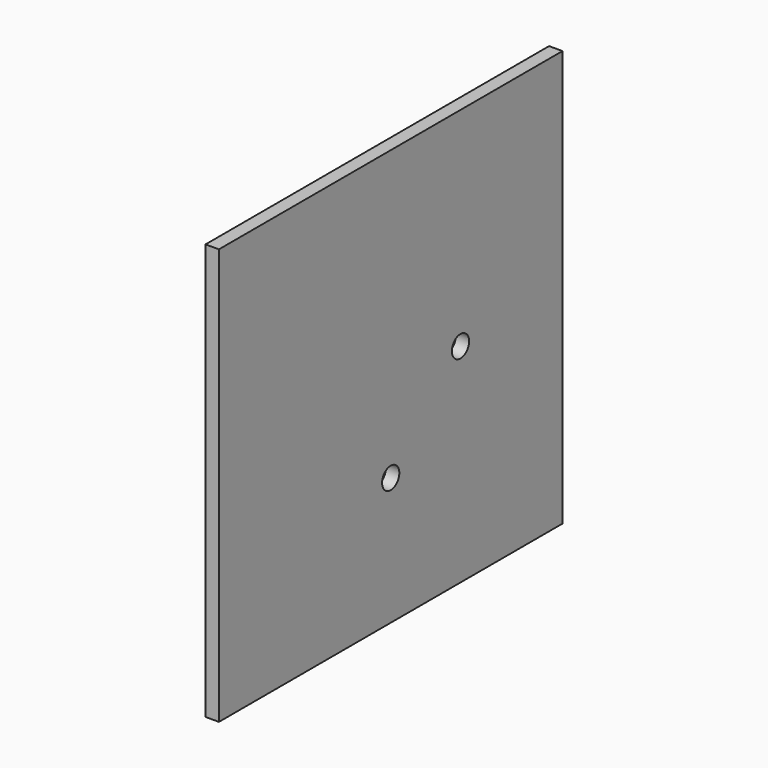
from build123d import *

# Parameters (mm, degrees)
F0_W     = 101.6
F0_H     = 98.425
F1_DEPTH = 3.175
F3_D     = 5.1054
F3_DEPTH = 25
F3_TIP   = 1.5338169022


# Not quite as in the source:
# - a length typed as a fraction of an inch, garbled in the dataset ("3 / 203.2 mm" for 3/8 in), is restored


with BuildPart() as f1:
    # F0 (on Right) → F1 (new body)
    with BuildSketch(Plane.YZ):
        Rectangle(F0_W, F0_H)
    extrude(amount=F1_DEPTH)

    # F3
    with Locations(Plane.YZ.offset(3.175)):
        with Locations((0, -19.05), (20.6375, 0)):
            Hole(F3_D / 2, depth=F3_DEPTH)
            with Locations((0, 0, -(F3_DEPTH + F3_TIP / 2))):  # 118° drill point
                Cone(0, F3_D / 2, F3_TIP, mode=Mode.SUBTRACT)


solid = f1.part
